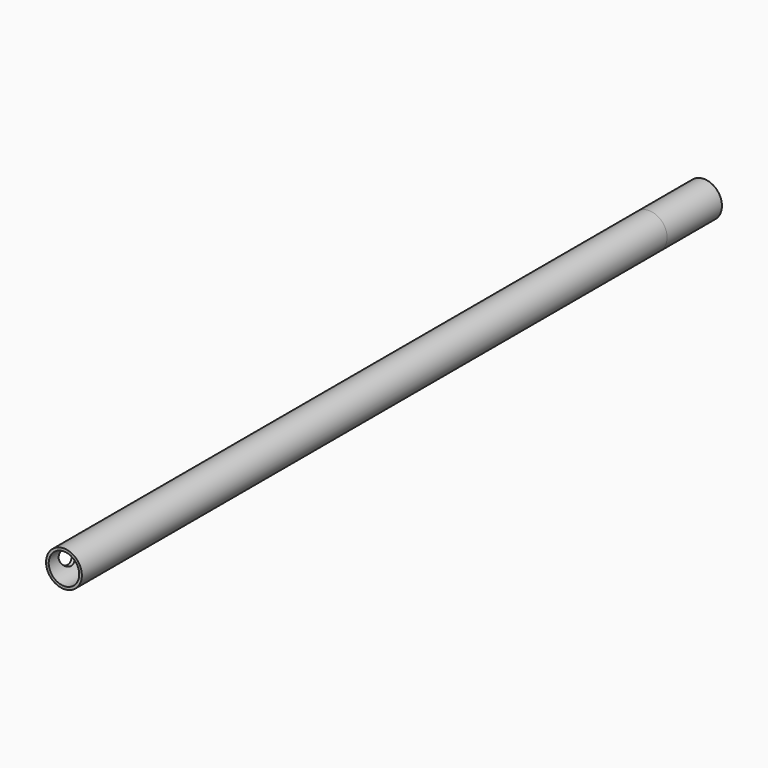
from build123d import *

# Parameters (mm, degrees)
F3_R      = 4.7
F4_DEPTH  = 167
F8_DEPTH  = 167
F6_R      = 4.7
F6_R_2    = 4
F9_DEPTH  = 25
F7_R      = 4.7
F7_R_2    = 4
F10_DEPTH = 18
F11_R     = 2.75
F12_DEPTH = 4.701


# Not quite as in the source:
# - ends of sketch curves that miss each other by under 0.0002 mm in the source are joined


with BuildPart() as f4:
    # F3 (on Front) → F4 (new body)
    with BuildSketch(Plane.XZ):
        Circle(F3_R)
    extrude(amount=F4_DEPTH)

    # F5 (on face) → F8 (cut, through all)
    with BuildSketch(Plane.XZ.offset(167)):
        with BuildLine():
            Line((-1.25, -3.8), (0, -3.8))
            Line((0, -3.8), (1.25, -3.8))
            Line((1.25, -3.8), (1.25, -3.7))
            ThreePointArc((1.25, -3.7), (1.3085786438, -3.5585786438), (1.45, -3.5))
            Line((1.45, -3.5), (2, -3.5))
            Line((2, -3.5), (2, -3.05))
            ThreePointArc((2, -3.05), (2.0585786438, -2.9085786438), (2.2, -2.85))
            Line((2.2, -2.85), (3.15, -2.85))
            Line((3.15, -2.85), (3.15, -2.15))
            Line((3.15, -2.15), (2.2, -2.15))
            ThreePointArc((2.2, -2.15), (2.0585786438, -2.0914213562), (2, -1.95))
            Line((2, -1.95), (2, -1.887459))
            ThreePointArc((2, -1.887459), (2.1033535752, -1.771554046), (2.2, -1.65))
            Line((2.2, -1.65), (3.75, -1.65))
            Line((3.75, -1.65), (3.75, 0))
            Line((3.75, 0), (3.75, 1.65))
            Line((3.75, 1.65), (2.2, 1.65))
            ThreePointArc((2.2, 1.65), (2.1033535752, 1.771554046), (1.9999998047, 1.8874588157))
            Line((1.9999998047, 1.8874588157), (2, 1.95))
            ThreePointArc((2, 1.95), (2.0585786438, 2.0914213562), (2.2, 2.15))
            Line((2.2, 2.15), (3.15, 2.15))
            Line((3.15, 2.15), (3.15, 2.85))
            Line((3.15, 2.85), (2.2, 2.85))
            ThreePointArc((2.2, 2.85), (2.0585786438, 2.9085786438), (2, 3.05))
            Line((2, 3.05), (2, 3.5))
            Line((2, 3.5), (1.45, 3.5))
            ThreePointArc((1.45, 3.5), (1.3085786438, 3.5585786438), (1.25, 3.7))
            Line((1.25, 3.7), (1.25, 3.8))
            Line((1.25, 3.8), (0, 3.8))
            Line((0, 3.8), (-1.25, 3.8))
            Line((-1.25, 3.8), (-1.25, 3.7))
            ThreePointArc((-1.25, 3.7), (-1.3085786438, 3.5585786438), (-1.45, 3.5))
            Line((-1.45, 3.5), (-2, 3.5))
            Line((-2, 3.5), (-2, 3.05))
            ThreePointArc((-2, 3.05), (-2.0585786438, 2.9085786438), (-2.2, 2.85))
            Line((-2.2, 2.85), (-3.15, 2.85))
            Line((-3.15, 2.85), (-3.15, 2.15))
            Line((-3.15, 2.15), (-2.2, 2.15))
            ThreePointArc((-2.2, 2.15), (-2.0585786438, 2.0914213562), (-2, 1.95))
            Line((-2, 1.95), (-2, 1.887459))
            ThreePointArc((-2, 1.887459), (-2.1033535752, 1.771554046), (-2.2, 1.65))
            Line((-2.2, 1.65), (-3.75, 1.65))
            Line((-3.75, 1.65), (-3.75, 0))
            Line((-3.75, 0), (-3.75, -1.65))
            Line((-3.75, -1.65), (-2.2, -1.65))
            ThreePointArc((-2.2, -1.65), (-2.1033535752, -1.771554046), (-1.9999998047, -1.8874588157))
            Line((-1.9999998047, -1.8874588157), (-2, -1.95))
            ThreePointArc((-2, -1.95), (-2.0585786438, -2.0914213562), (-2.2, -2.15))
            Line((-2.2, -2.15), (-3.15, -2.15))
            Line((-3.15, -2.15), (-3.15, -2.85))
            Line((-3.15, -2.85), (-2.2, -2.85))
            ThreePointArc((-2.2, -2.85), (-2.0585786438, -2.9085786438), (-2, -3.05))
            Line((-2, -3.05), (-2, -3.5))
            Line((-2, -3.5), (-1.45, -3.5))
            ThreePointArc((-1.45, -3.5), (-1.3085786438, -3.5585786438), (-1.25, -3.7))
            Line((-1.25, -3.7), (-1.25, -3.8))
        make_face()
    extrude(amount=-F8_DEPTH, mode=Mode.SUBTRACT)

    # F6 (on face) → F9 (join)
    with BuildSketch(Plane.XZ.offset(167)):
        Circle(F6_R)
        Circle(F6_R_2, mode=Mode.SUBTRACT)
    extrude(amount=F9_DEPTH)

    # F7 (on face) → F10 (join)
    with BuildSketch(Plane(origin=(0, 0, 0), x_dir=(-1, 0, 0), z_dir=(0, 1, 0))):
        Circle(F7_R)
        Circle(F7_R_2, mode=Mode.SUBTRACT)
    extrude(amount=F10_DEPTH)

    # F11 (on Right) → F12 (cut, through all)
    with BuildSketch(Plane.YZ):
        with Locations((-186, 0)):
            Circle(F11_R)
    extrude(amount=-F12_DEPTH, mode=Mode.SUBTRACT)


solid = f4.part
